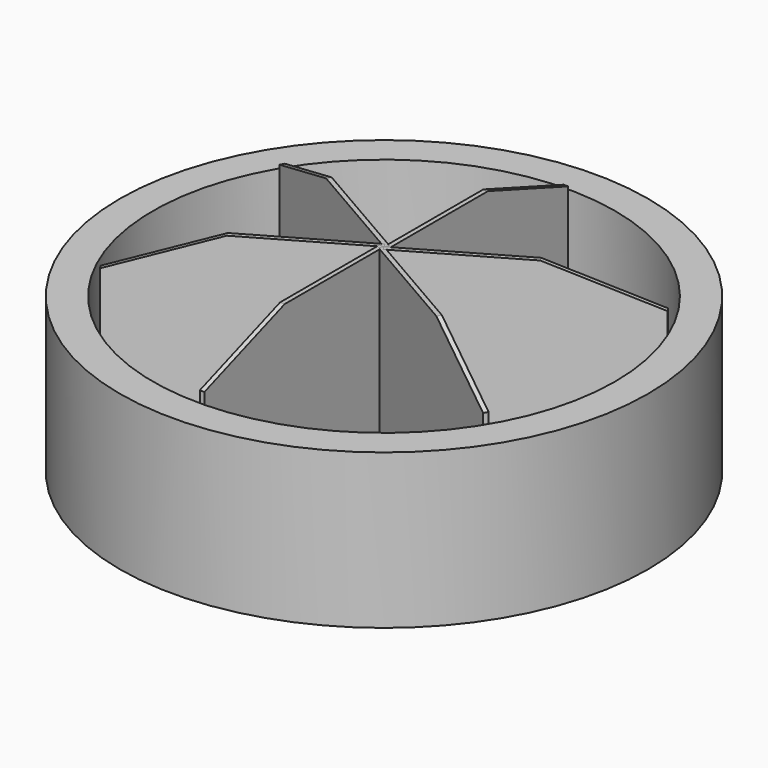
from build123d import *

# Parameters (mm, degrees)
F0_R     = 101.6
F1_DEPTH = 59.436
F2_R     = 88.9
F3_DEPTH = 56.388
F5_DEPTH = 1.778
F6_COUNT = 6


# Not quite as in the source:
# - the program builds the solid bodies; features that only make, move or delete a surface that nothing else refers to are left out


with BuildPart() as f1:
    # F0 (on Top) → F1 (new body)
    with BuildSketch(Plane.XY):
        Circle(F0_R)
    extrude(amount=F1_DEPTH)

    # F2 (on face) → F3 (cut)
    with BuildSketch(Plane.XY.offset(59.436)):
        Circle(F2_R)
    extrude(amount=-F3_DEPTH, mode=Mode.SUBTRACT)


with BuildPart() as f5:
    # F4 (on Right) → F5 (new body)
    with BuildSketch(Plane.YZ):
        Polygon((0, 6.9354507141), (76.844625175, 6.4341924153), (86.36, 18.4533931315), (86.36, 62.1109679341), (47.7517807697, 76.2), (0, 76.2), align=None)
    extrude(amount=F5_DEPTH)


with BuildPart() as f6_1:
    # F6: instance of F5
    add(f5.part.rotate(Axis((0, 0, 59.436), (0, 0, 1)), 1 * 360 / F6_COUNT))


with BuildPart() as f6_2:
    # F6: instance of F5
    add(f5.part.rotate(Axis((0, 0, 59.436), (0, 0, 1)), 2 * 360 / F6_COUNT))


with BuildPart() as f6_3:
    # F6: instance of F5
    add(f5.part.rotate(Axis((0, 0, 59.436), (0, 0, 1)), 3 * 360 / F6_COUNT))


with BuildPart() as f6_4:
    # F6: instance of F5
    add(f5.part.rotate(Axis((0, 0, 59.436), (0, 0, 1)), 4 * 360 / F6_COUNT))


with BuildPart() as f6_5:
    # F6: instance of F5
    add(f5.part.rotate(Axis((0, 0, 59.436), (0, 0, 1)), 5 * 360 / F6_COUNT))


solid = Compound([f1.part, f5.part, f6_1.part, f6_2.part, f6_3.part, f6_4.part, f6_5.part])
